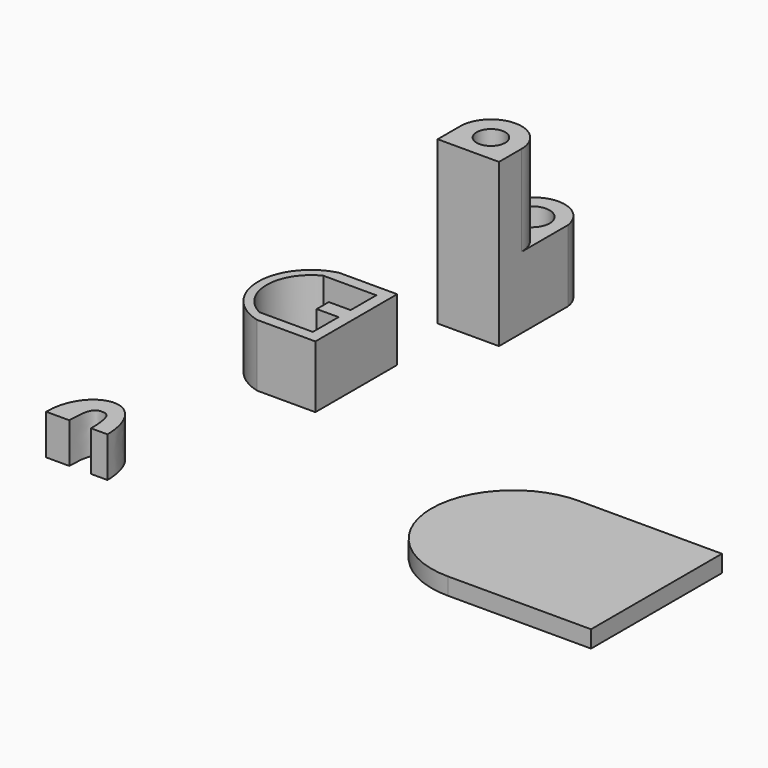
from build123d import *

# Parameters (mm, degrees)
F1_DEPTH = 2.5
F3_DEPTH = 9.14
F5_DEPTH = 5.9
F7_R     = 2.1
F8_DEPTH = 23.8
F7_R_2   = 2.6
F9_DEPTH = 10.5


# Not quite as in the source:
# - a feature names something its author has since deleted; it is built from what else it names


with BuildPart() as f1:
    # F0 (on Top) → F1 (new body)
    with BuildSketch(Plane.XY):
        with BuildLine():
            Line((32.6696708798, -0.8768981546), (11.6696708798, -0.8768981546))
            ThreePointArc((11.6696708798, -0.8768981546), (-0.3303291202, -12.8768981546), (11.6696708798, -24.8768981546))
            Line((11.6696708798, -24.8768981546), (32.6696708798, -24.8768981546))
            Line((32.6696708798, -24.8768981546), (32.6696708798, -0.8768981546))
        make_face()
    extrude(amount=F1_DEPTH)


with BuildPart() as f3:
    # F2 (on Top) → F3 (new body)
    with BuildSketch(Plane.XY):
        with BuildLine():
            Line((-28.6330851495, 16.2008921671), (-37.1832723155, 16.2008921671))
            ThreePointArc((-37.1832723155, 16.2008921671), (-43.0276089021, 8.7008921671), (-37.1832723155, 1.2008921671))
            Line((-37.1832723155, 1.2008921671), (-28.6330851495, 1.2008921671))
            Line((-28.6330851495, 1.2008921671), (-28.6330851495, 16.2008921671))
        make_face()
        with BuildLine():
            Line((-32.4330851495, 7.5708921671), (-31.3330851495, 7.5708921671))
            Line((-31.3330851495, 7.5708921671), (-30.3330851495, 7.5708921671))
            Line((-30.3330851495, 7.5708921671), (-30.3330851495, 2.8584186471))
            Line((-30.3330851495, 2.8584186471), (-36.8416506207, 2.8584186471))
            Line((-36.8416506207, 2.8584186471), (-38.1814390978, 2.8584186471))
            ThreePointArc((-38.1814390978, 2.8584186471), (-41.7566770007, 8.7022804581), (-38.1085063391, 14.5008921671))
            Line((-38.1085063391, 14.5008921671), (-36.8416506207, 14.5008921671))
            Line((-36.8416506207, 14.5008921671), (-30.3330851495, 14.5008921671))
            Line((-30.3330851495, 14.5008921671), (-30.3330851495, 9.7884186471))
            Line((-30.3330851495, 9.7884186471), (-31.3330851495, 9.7884186471))
            Line((-31.3330851495, 9.7884186471), (-33.5330851495, 9.7884186471))
            Line((-33.5330851495, 9.7884186471), (-33.5330851495, 8.7008921671))
            Line((-33.5330851495, 8.7008921671), (-33.5330851495, 7.5708921671))
            Line((-33.5330851495, 7.5708921671), (-32.4330851495, 7.5708921671))
        make_face(mode=Mode.SUBTRACT)
    extrude(amount=F3_DEPTH)


with BuildPart() as f5:
    # F4 (on Top) → F5 (new body)
    with BuildSketch(Plane.XY):
        with BuildLine():
            Line((-39.1227118313, -26.8252976239), (-36.7227118313, -26.8252976239))
            add(Edge.make_bspline(
                [(-45.7227118313, -26.8252976239), (-45.7227118313, -22.374657914), (-40.3570640003, -17.7727615296), (-36.7684476078, -22.9574795812), (-36.7227118313, -26.8252976239)],
                knots=[0, 0, 0, 0, 0.5087944096, 1, 1, 1, 1], degree=3))
            Line((-45.7227118313, -26.8252976239), (-42.3227118313, -26.8252976239))
            add(Edge.make_bspline(
                [(-42.3227118313, -26.8252976239), (-42.3142164946, -22.9051690549), (-40.695380196, -22.7360589504), (-39.1858704388, -22.9239035398), (-39.1227118313, -26.8252976239)],
                knots=[0, 0, 0, 0, 0.5, 1, 1, 1, 1], degree=3))
        make_face()
    extrude(amount=F5_DEPTH)


with BuildPart() as f6_1:
    # F6: copy of F5
    add(f5.part)


with BuildPart() as f8:
    # F7 (on Top) → F8 (new body)
    with BuildSketch(Plane.XY):
        with BuildLine():
            ThreePointArc((-31.441547364, 31.2786275238), (-30.6885375354, 28.7866273922), (-28.6815186281, 27.1286275238))
            Line((-28.6815186281, 27.1286275238), (-25.2015760999, 27.1286275238))
            ThreePointArc((-25.2015760999, 27.1286275238), (-23.1945571926, 28.7866273922), (-22.441547364, 31.2786275238))
            ThreePointArc((-22.441547364, 31.2786275238), (-26.941547364, 35.7786275238), (-31.441547364, 31.2786275238))
        make_face()
        with Locations((-26.941547364, 31.2786275238)):
            Circle(F7_R, mode=Mode.SUBTRACT)
        with BuildLine():
            Line((-31.441547364, 31.2786275238), (-31.441547364, 27.1286275238))
            Line((-31.441547364, 27.1286275238), (-28.6815186281, 27.1286275238))
            ThreePointArc((-28.6815186281, 27.1286275238), (-30.6885375354, 28.7866273922), (-31.441547364, 31.2786275238))
        make_face()
        with BuildLine():
            ThreePointArc((-22.441547364, 31.2786275238), (-23.1945571926, 28.7866273922), (-25.2015760999, 27.1286275238))
            Line((-25.2015760999, 27.1286275238), (-22.441547364, 27.1286275238))
            Line((-22.441547364, 27.1286275238), (-22.441547364, 31.2786275238))
        make_face()
    extrude(amount=F8_DEPTH)

    # F7 (on Top) → F9 (join)
    with BuildSketch(Plane.XY):
        with BuildLine():
            Line((-31.441547364, 39.8286275238), (-31.441547364, 31.2786275238))
            ThreePointArc((-31.441547364, 31.2786275238), (-26.941547364, 35.7786275238), (-22.441547364, 31.2786275238))
            Line((-22.441547364, 31.2786275238), (-22.441547364, 39.8286275238))
            ThreePointArc((-22.441547364, 39.8286275238), (-26.941547364, 43.6803370595), (-31.441547364, 39.8286275238))
        make_face()
        with Locations((-26.941547364, 38.7973775238)):
            Circle(F7_R_2, mode=Mode.SUBTRACT)
    extrude(amount=F9_DEPTH)


solid = Compound([f1.part, f3.part, f5.part, f6_1.part, f8.part])
